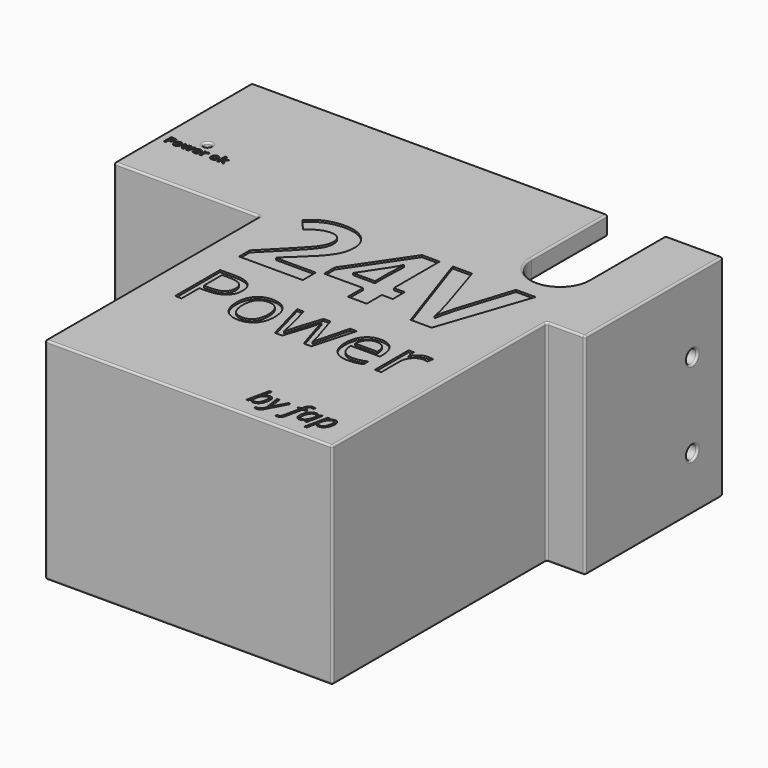
from build123d import *

# Parameters (mm, degrees)
F0_R            = 1
F1_DEPTH        = 5
F2_W            = 65
F2_H            = 50
F2_H_2          = 5
F3_DEPTH        = 5
F4_W            = 43
F4_H            = 50
F4_H_2          = 5
F5_DEPTH        = 5
F6_W            = 15
F6_H            = 5
F6_H_2          = 50
F7_DEPTH        = 5
F8_W            = 40
F8_H            = 50
F8_R            = 1.75
F9_DEPTH        = 5
F10_W           = 47
F10_H           = 27
F11_DEPTH       = 5
F12_W           = 40
F12_H           = 50
F12_R           = 1.75
F13_DEPTH       = 5
F14_W           = 65
F14_H           = 50
F15_DEPTH       = 5
F16_TEXT_SIZE   = 33.3333333333
F16_TEXT_SIZE_2 = 7.8242284416
F16_TEXT_SIZE_3 = 20.5981794538
F16_TEXT_SIZE_4 = 3.4722222222
F17_DEPTH       = 0.5
F18_R           = 0.5


# Not quite as in the source:
# - Text() gives the source's letters only with a copy of the font that has no kerning and outlines rounded to 1/6400 em; it was checked with that copy


with BuildPart() as f1:
    # F0 (on Top) → F1 (new body)
    with BuildSketch(Plane.XY):
        with BuildLine():
            Line((31.5, 61.5484006821), (-61.5, 61.5484006821))
            Line((-61.5, 61.5484006821), (-61.5, 16.5484006821))
            Line((-61.5, 16.5484006821), (-18.5, 16.5484006821))
            Line((-18.5, 16.5484006821), (-18.5, -48.4515993179))
            Line((-18.5, -48.4515993179), (46.5, -48.4515993179))
            Line((46.5, -48.4515993179), (46.5, 16.5484006821))
            Line((46.5, 16.5484006821), (61.5, 16.5484006821))
            Line((61.5, 16.5484006821), (61.5, 61.5484006821))
            Line((61.5, 61.5484006821), (46.5, 61.5484006821))
            Line((46.5, 61.5484006821), (46.5, 36.5484006821))
            ThreePointArc((46.5, 36.5484006821), (39, 29.0484006821), (31.5, 36.5484006821))
            Line((31.5, 36.5484006821), (31.5, 61.5484006821))
        make_face()
        with Locations((-51.5, 34.5484006821)):
            Circle(F0_R, mode=Mode.SUBTRACT)
    extrude(amount=-F1_DEPTH)

    # F2 (on face) → F3 (join)
    with BuildSketch(Plane.XZ.offset(48.4515993179)):
        with Locations((14, -30)):
            Rectangle(F2_W, F2_H)
        with Locations((14, -2.5)):
            Rectangle(F2_W, F2_H_2)
    extrude(amount=F3_DEPTH)

    # F4 (on face) → F5 (join)
    with BuildSketch(Plane.XZ.offset(-16.5484006821)):
        with Locations((-40, -30)):
            Rectangle(F4_W, F4_H)
        with Locations((-40, -2.5)):
            Rectangle(F4_W, F4_H_2)
    extrude(amount=-F5_DEPTH)

    # F6 (on face) → F7 (join)
    with BuildSketch(Plane.XZ.offset(-16.5484006821)):
        with Locations((54, -2.5)):
            Rectangle(F6_W, F6_H)
        with Locations((54, -30)):
            Rectangle(F6_W, F6_H_2)
    extrude(amount=-F7_DEPTH)

    # F8 (on face) → F9 (join)
    with BuildSketch(Plane(origin=(-61.5, 0, 0), x_dir=(0, -1, 0), z_dir=(-1, 0, 0))):
        with Locations((-41.5484006821, -30)):
            Rectangle(F8_W, F8_H)
        with Locations((-51.5484006821, -41)):
            Circle(F8_R, mode=Mode.SUBTRACT)
        with Locations((-51.5484006821, -19)):
            Circle(F8_R, mode=Mode.SUBTRACT)
        Polygon((-16.5484006821, 0), (-61.5484006821, 0), (-61.5484006821, -5), (-21.5484006821, -5), (-21.5484006821, -55), (-16.5484006821, -55), align=None)
    extrude(amount=-F9_DEPTH)

    # F10 (on face) → F11 (join)
    with BuildSketch(Plane(origin=(-18.5, 0, 0), x_dir=(0, -1, 0), z_dir=(-1, 0, 0))):
        Polygon((53.4515993179, 0), (-16.5484006821, 0), (-16.5484006821, -5), (48.4515993179, -5), (48.4515993179, -55), (53.4515993179, -55), align=None)
        with BuildLine():
            Line((48.4515993179, -5), (-16.5484006821, -5))
            Line((-16.5484006821, -5), (-16.5484006821, -55))
            Line((-16.5484006821, -55), (-11.5484006821, -55))
            ThreePointArc((-11.5484006821, -55), (-4.0484006821, -47.5), (3.4515993179, -55))
            Line((3.4515993179, -55), (48.4515993179, -55))
            Line((48.4515993179, -55), (48.4515993179, -5))
        make_face()
        with Locations((21.5132973492, -30)):
            Rectangle(F10_W, F10_H, mode=Mode.SUBTRACT)
    extrude(amount=F11_DEPTH)

    # F12 (on face) → F13 (join)
    with BuildSketch(Plane.YZ.offset(61.5)):
        with Locations((41.5484006821, -30)):
            Rectangle(F12_W, F12_H)
        with Locations((51.5484006821, -41)):
            Circle(F12_R, mode=Mode.SUBTRACT)
        with Locations((51.5484006821, -19)):
            Circle(F12_R, mode=Mode.SUBTRACT)
        Polygon((16.5484006821, 0), (16.5484006821, -55), (21.5484006821, -55), (21.5484006821, -5), (61.5484006821, -5), (61.5484006821, 0), align=None)
    extrude(amount=-F13_DEPTH)

    # F14 (on face) → F15 (join)
    with BuildSketch(Plane.YZ.offset(46.5)):
        with Locations((-15.9515993179, -30)):
            Rectangle(F14_W, F14_H)
        Polygon((-53.4515993179, 0), (-53.4515993179, -55), (-48.4515993179, -55), (-48.4515993179, -5), (16.5484006821, -5), (16.5484006821, 0), align=None)
    extrude(amount=F15_DEPTH)

    # F16 (on face) → F17 (cut)
    with BuildSketch(Plane.XY):
        with Locations((-16.9375, 0)):
            Text('24V', F16_TEXT_SIZE, font='Open Sans', font_style=FontStyle.BOLD, text_align=(TextAlign.LEFT, TextAlign.BOTTOM))
        with Locations((24.8305548238, -48.4515993179)):
            Text('by fap', F16_TEXT_SIZE_2, font='Open Sans', font_style=FontStyle.ITALIC, text_align=(TextAlign.LEFT, TextAlign.BOTTOM))
        with Locations((-16.9375, -21.7631865609)):
            Text('Power', F16_TEXT_SIZE_3, font='Open Sans', text_align=(TextAlign.LEFT, TextAlign.BOTTOM))
        with Locations((-59.680609809, 30.0484006821)):
            Text('Power ok', F16_TEXT_SIZE_4, font='Open Sans', font_style=FontStyle.BOLD, text_align=(TextAlign.LEFT, TextAlign.BOTTOM))
    extrude(amount=-F17_DEPTH, mode=Mode.SUBTRACT)

    # F18
    f18_edges = [f1.edges().sort_by_distance(p)[0] for p in [
        (14, -53.451599, 0),
        (51.5, -18.451599, 0),
        (56.5, 16.548401, 0),
        (61.5, 39.048401, 0),
        (61.5, 16.548401, -27.5),
        (51.5, 16.548401, -27.5),
        (51.5, -53.451599, -27.5),
        (51.5, -18.451599, -55),
        (14, -53.451599, -55),
        (56.5, 16.548401, -55),
        (61.5, 39.048401, -55),
        (61.5, 49.798401, -41),
        (61.5, 49.798401, -19),
        (61.5, 61.548401, -27.5),
        (54, 61.548401, 0),
        (46.5, 49.048401, 0),
        (39, 29.048401, 0),
        (31.5, 49.048401, 0),
        (-15, 61.548401, 0),
        (-61.5, 39.048401, 0),
        (-42.5, 16.548401, 0),
        (-23.5, -18.451599, 0),
        (-61.5, 16.548401, -27.5),
        (-23.5, -53.451599, -27.5),
        (-23.5, 16.548401, -27.5),
        (-61.5, 53.298401, -19),
        (-61.5, 53.298401, -41),
        (-61.5, 61.548401, -27.5),
        (-61.5, 39.048401, -55),
        (-42.5, 16.548401, -55),
        (-23.5, -21.513297, -43.5),
        (-23.5, 1.986703, -30),
        (-23.5, -45.013297, -30),
        (-23.5, -21.513297, -16.5),
        (-23.5, -28.451599, -55),
        (-23.5, 4.048401, -47.5),
        (-23.5, 14.048401, -55),
        (-18.5, -25.951599, -55),
        (-18.5, 4.048401, -47.5),
        (-18.5, 16.548401, -55),
        (-37.5, 21.548401, -55),
        (-56.5, 41.548401, -55),
        (-56.5, 61.548401, -30),
        (-12.5, 61.548401, -5),
        (46.5, 61.548401, -2.5),
        (46.5, 49.048401, -5),
        (39, 29.048401, -5),
        (31.5, 49.048401, -5),
        (-59, 61.548401, -55),
        (59, 61.548401, -55),
        (-21, -3.451599, -55),
        (-21, 11.548401, -55),
        (-18.5, 1.986703, -30),
        (-18.5, -21.513297, -16.5),
        (-18.5, -21.513297, -43.5),
        (-18.5, -45.013297, -30),
        (56.5, 49.798401, -41),
        (56.5, 49.798401, -19),
        (56.5, 41.548401, -55),
        (51.5, 21.548401, -55),
        (46.5, -13.451599, -55),
        (14, -48.451599, -55),
        (-56.5, 53.298401, -41),
        (-56.5, 53.298401, -19),
        (-52.5, 34.548401, -5),
        (-18.5, 21.548401, -30),
        (-52.5, 34.548401, 0),
        (46.5, 21.548401, -30),
        (31.5, 61.548401, -2.5),
        (56.5, 61.548401, -30),
        (51.5, 61.548401, -5),
    ]]
    fillet(f18_edges, radius=F18_R)


solid = f1.part
